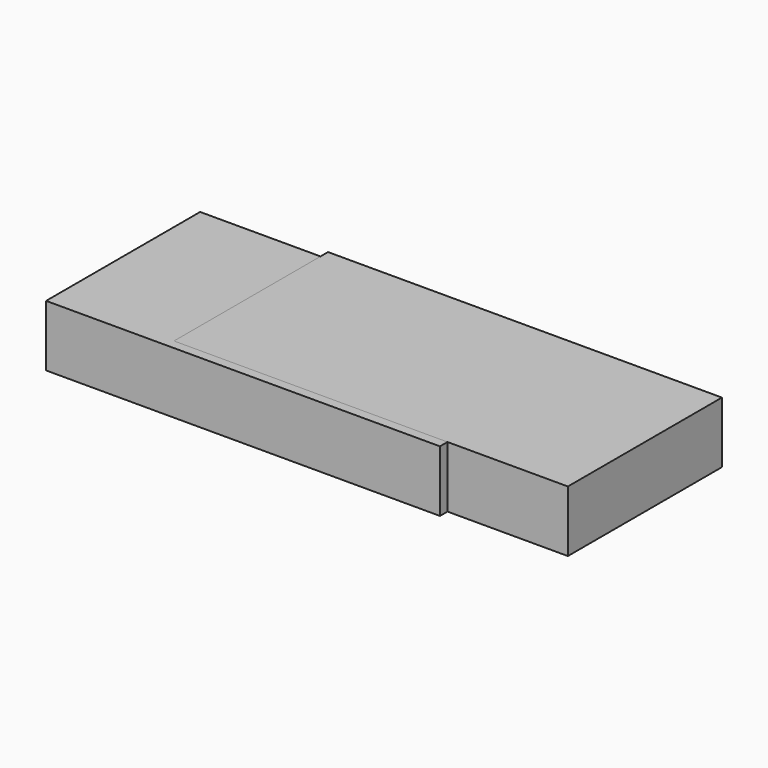
from build123d import *

# Parameters (mm, degrees)
F0_W     = 114.3
F0_H     = 55.88
F1_DEPTH = 10.16
F2_W     = 114.3
F2_H     = 55.88
F3_DEPTH = 17.78
F4_T     = -6.35
F5_T     = -6.35


with BuildPart() as f1:
    # F0 (on Top) → F1 (new body)
    with BuildSketch(Plane.XY):
        with Locations((0.5737692118, -14.1728672351)):
            Rectangle(F0_W, F0_H)
    extrude(amount=F1_DEPTH)

    # F5
    f5_openings = [f1.faces().sort_by_distance(p)[0] for p in [
        (0.573769, -14.172867, 10.16),
    ]]
    offset(amount=F5_T, openings=f5_openings)


with BuildPart() as f3:
    # F2 (on Top) → F3 (new body)
    with BuildSketch(Plane.XY):
        with Locations((-34.3610338222, -16.905572731)):
            Rectangle(F2_W, F2_H)
    extrude(amount=F3_DEPTH)

    # F4
    f4_openings = [f3.faces().sort_by_distance(p)[0] for p in [
        (-34.361034, -16.905573, 0),
    ]]
    offset(amount=F4_T, openings=f4_openings)


with BuildPart() as f3b:
    # F0 (on Top) → F3, piece 2 (new body)
    with BuildSketch(Plane.XY):
        with Locations((0.5737692118, -14.1728672351)):
            Rectangle(F0_W, F0_H)
    extrude(amount=F3_DEPTH)


solid = Compound([f1.part, f3.part, f3b.part])
